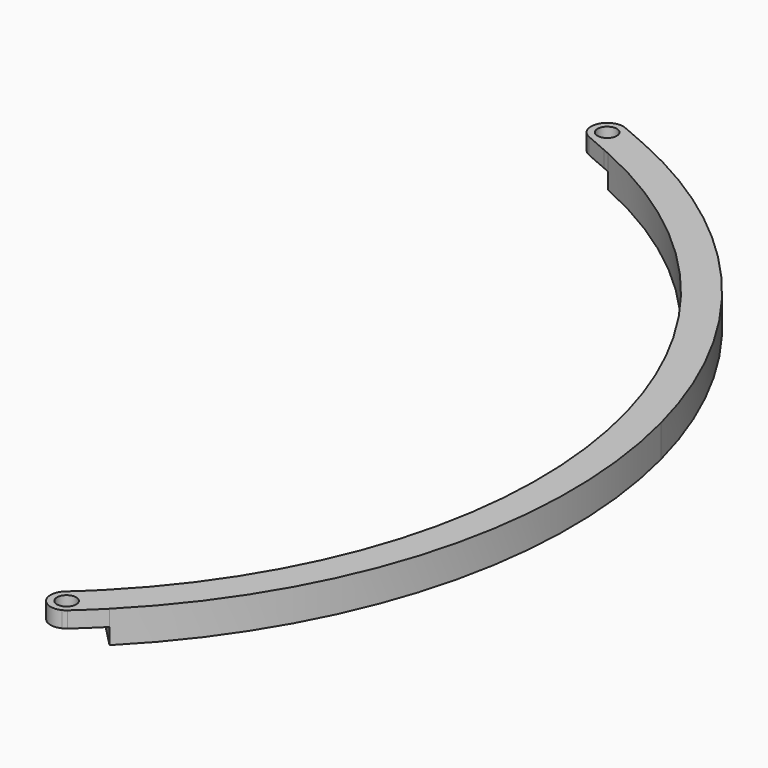
from build123d import *

# Parameters (mm, degrees)
F0_R     = 1.5
F1_DEPTH = 5
F2_DEPTH = 2.5
F4_DEPTH = 2.5


# Not quite as in the source:
# - a feature names something its author has since deleted; it is built from what else it names


with BuildPart() as f1:
    # F0 (on Top) → F1 (new body)
    with BuildSketch(Plane.XY):
        with BuildLine():
            Line((30, 51.9615242271), (32.4836596815, 56.2633489842))
            Line((32.4836596815, 56.2633489842), (28.4224519805, 58.0264243292))
            ThreePointArc((28.4224519805, 58.0264243292), (25.1336779708, 56.7287473614), (26.4313549386, 53.4399733516))
            Line((26.4313549386, 53.4399733516), (29.967319363, 51.9049197034))
            Line((29.967319363, 51.9049197034), (30, 51.9615242271))
        make_face()
        with Locations((27.4269034596, 55.7331988404)):
            Circle(F0_R, mode=Mode.SUBTRACT)
        with BuildLine():
            ThreePointArc((67.5061883913, 18.5179515304), (63.7494272333, 28.9138466382), (58.4029909795, 38.5887372772))
            ThreePointArc((58.4029909795, 38.5887372772), (46.511709986, 48.4848469682), (33.0089029581, 56.0353272873))
            Line((33.0089029581, 56.0353272873), (31.0178059162, 51.4488763097))
            ThreePointArc((31.0178059162, 51.4488763097), (51.8847287198, 37.8894735935), (67.5061883913, 18.5179515304))
        make_face()
        Polygon((31.0178059162, 51.4488763097), (33.0089029581, 56.0353272873), (32.4836596815, 56.2633489842), (30, 51.9615242271), (29.967319363, 51.9049197034), align=None)
        with BuildLine():
            ThreePointArc((54.2641944404, -83.9964118384), (54.5449950566, -83.8143395504), (54.8251847727, -83.6313285476))
            ThreePointArc((54.8251847727, -83.6313285476), (56.7197095597, -81.8911804241), (58.5601267726, -80.0939035554))
            Line((58.5601267726, -80.0939035554), (55.0705599201, -76.5129397591))
            ThreePointArc((55.0705599201, -76.5129397591), (53.341493873, -78.2050105238), (51.5614910891, -79.8434130866))
            ThreePointArc((51.5614910891, -79.8434130866), (51.0979794421, -83.1009956935), (54.2641944404, -83.9964118384))
        make_face()
        with Locations((53.1933379309, -81.7373708171)):
            Circle(F0_R, mode=Mode.SUBTRACT)
        with BuildLine():
            Line((55.0705599201, -76.5129397591), (58.5601267726, -80.0939035554))
            ThreePointArc((58.5601267726, -80.0939035554), (80.0342840094, -42.9250014233), (80.3674019431, 0))
            Line((80.3674019431, 0), (75.1959644791, 0))
            ThreePointArc((75.1959644791, 0), (75.3863719236, -40.9533729371), (55.0705599201, -76.5129397591))
        make_face()
        with BuildLine():
            ThreePointArc((54.2641944404, -83.9964118384), (54.5569628073, -83.8327293059), (54.8251847727, -83.6313285476))
            ThreePointArc((54.8251847727, -83.6313285476), (54.5449950566, -83.8143395504), (54.2641944404, -83.9964118384))
        make_face()
        with BuildLine():
            Line((75.1959644791, 0), (80.3674019431, 0))
            ThreePointArc((80.3674019431, 0), (71.977896021, 20.7701131861), (58.4029909795, 38.5887372772))
            ThreePointArc((58.4029909795, 38.5887372772), (63.7494272333, 28.9138466382), (67.5061883913, 18.5179515304))
            ThreePointArc((67.5061883913, 18.5179515304), (71.9402181457, 9.5036231189), (75.1959644791, 0))
        make_face()
    extrude(amount=F1_DEPTH)


with BuildPart() as f2:
    # F0 (on Top) → F2 (new body)
    with BuildSketch(Plane.XY):
        Polygon((31.0178059162, 51.4488763097), (33.0089029581, 56.0353272873), (32.4836596815, 56.2633489842), (30, 51.9615242271), (29.967319363, 51.9049197034), align=None)
        with BuildLine():
            Line((30, 51.9615242271), (32.4836596815, 56.2633489842))
            Line((32.4836596815, 56.2633489842), (28.4224519805, 58.0264243292))
            ThreePointArc((28.4224519805, 58.0264243292), (25.1336779708, 56.7287473614), (26.4313549386, 53.4399733516))
            Line((26.4313549386, 53.4399733516), (29.967319363, 51.9049197034))
            Line((29.967319363, 51.9049197034), (30, 51.9615242271))
        make_face()
        with Locations((27.4269034596, 55.7331988404)):
            Circle(F0_R, mode=Mode.SUBTRACT)
    extrude(amount=F2_DEPTH)


with BuildPart() as f1_1:
    add(f1.part)

    # F3: cut F2
    add(f2.part, mode=Mode.SUBTRACT)


with BuildPart() as f4:
    # F0 (on Top) → F4 (new body)
    with BuildSketch(Plane.XY):
        with BuildLine():
            ThreePointArc((54.2641944404, -83.9964118384), (54.5449950566, -83.8143395504), (54.8251847727, -83.6313285476))
            ThreePointArc((54.8251847727, -83.6313285476), (56.7197095597, -81.8911804241), (58.5601267726, -80.0939035554))
            Line((58.5601267726, -80.0939035554), (55.0705599201, -76.5129397591))
            ThreePointArc((55.0705599201, -76.5129397591), (53.341493873, -78.2050105238), (51.5614910891, -79.8434130866))
            ThreePointArc((51.5614910891, -79.8434130866), (51.0979794421, -83.1009956935), (54.2641944404, -83.9964118384))
        make_face()
        with Locations((53.1933379309, -81.7373708171)):
            Circle(F0_R, mode=Mode.SUBTRACT)
        with BuildLine():
            ThreePointArc((54.2641944404, -83.9964118384), (54.5569628073, -83.8327293059), (54.8251847727, -83.6313285476))
            ThreePointArc((54.8251847727, -83.6313285476), (54.5449950566, -83.8143395504), (54.2641944404, -83.9964118384))
        make_face()
    extrude(amount=F4_DEPTH)


with BuildPart() as f1_2:
    add(f1_1.part)

    # F5: cut F4
    add(f4.part, mode=Mode.SUBTRACT)


solid = f1_2.part
